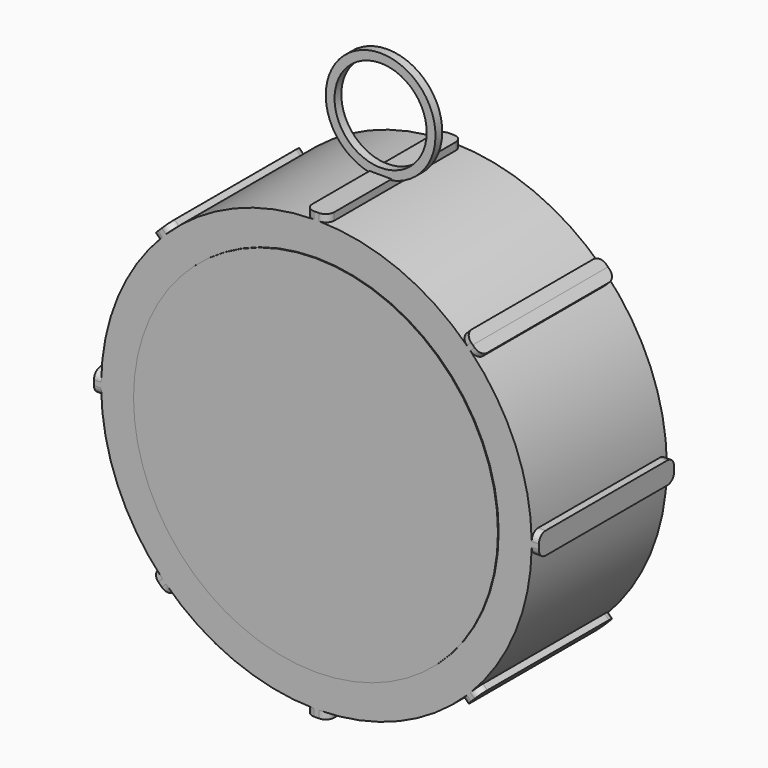
from build123d import *

# Parameters (mm, degrees)
F0_R     = 32.3708711279
F1_DEPTH = 12.7
F2_R     = 27.3986132433
F3_DEPTH = 12.827
F5_DEPTH = 25.4
F6_R     = 1.27
F8_R     = 8.2490124286
F8_R_2   = 6.9276952265
F9_DEPTH = 0.635


# Not quite as in the source:
# - two fillets or chamfers of one size are made in one step


with BuildPart() as f1:
    # F0 (on Front) → F1 (new body, symmetric)
    with BuildSketch(Plane.XZ):
        Circle(F0_R)
    extrude(amount=F1_DEPTH, both=True)

    # F2 (on Front) → F3 (join, symmetric)
    with BuildSketch(Plane.XZ):
        Circle(F2_R)
    extrude(amount=F3_DEPTH, both=True)

    # F4 (on face) → F5 (join)
    with BuildSketch(Plane.XZ.offset(12.7)):
        with BuildLine():
            ThreePointArc((-24.0273053052, 21.6924387138), (-22.8896624875, 22.8896624875), (-21.6924387138, 24.0273053052))
            Line((-21.6924387138, 24.0273053052), (-22.3403787647, 24.6752453562))
            Line((-22.3403787647, 24.6752453562), (-23.5078120604, 23.5078120604))
            Line((-23.5078120604, 23.5078120604), (-24.6752453562, 22.3403787647))
            Line((-24.6752453562, 22.3403787647), (-24.0273053052, 21.6924387138))
        make_face()
        with BuildLine():
            Line((24.6752453562, 22.3403787647), (23.5078120604, 23.5078120604))
            Line((23.5078120604, 23.5078120604), (22.3403787647, 24.6752453562))
            Line((22.3403787647, 24.6752453562), (21.6924387138, 24.0273053052))
            ThreePointArc((21.6924387138, 24.0273053052), (22.8896624875, 22.8896624875), (24.0273053052, 21.6924387138))
            Line((24.0273053052, 21.6924387138), (24.6752453562, 22.3403787647))
        make_face()
        with BuildLine():
            Line((24.6752453562, -22.3403787647), (24.0273053052, -21.6924387138))
            ThreePointArc((24.0273053052, -21.6924387138), (22.8896624875, -22.8896624875), (21.6924387138, -24.0273053052))
            Line((21.6924387138, -24.0273053052), (22.3403787647, -24.6752453562))
            Line((22.3403787647, -24.6752453562), (23.5078120604, -23.5078120604))
            Line((23.5078120604, -23.5078120604), (24.6752453562, -22.3403787647))
        make_face()
        with BuildLine():
            ThreePointArc((-21.6924387138, -24.0273053052), (-22.8896624875, -22.8896624875), (-24.0273053052, -21.6924387138))
            Line((-24.0273053052, -21.6924387138), (-24.6752453562, -22.3403787647))
            Line((-24.6752453562, -22.3403787647), (-23.5078120604, -23.5078120604))
            Line((-23.5078120604, -23.5078120604), (-22.3403787647, -24.6752453562))
            Line((-22.3403787647, -24.6752453562), (-21.6924387138, -24.0273053052))
        make_face()
        with BuildLine():
            Line((1.651, -33.4515422583), (1.651, -32.3287410299))
            ThreePointArc((1.651, -32.3287410299), (0, -32.3708711279), (-1.651, -32.3287410299))
            Line((-1.651, -32.3287410299), (-1.651, -33.4515422583))
            Line((-1.651, -33.4515422583), (0, -33.4515422583))
            Line((0, -33.4515422583), (1.651, -33.4515422583))
        make_face()
        with BuildLine():
            ThreePointArc((-32.3287410299, -1.651), (-32.3708711279, 0), (-32.3287410299, 1.651))
            Line((-32.3287410299, 1.651), (-33.4515480299, 1.651))
            Line((-33.4515480299, 1.651), (-33.4515480299, 0))
            Line((-33.4515480299, 0), (-33.4515480299, -1.651))
            Line((-33.4515480299, -1.651), (-32.3287410299, -1.651))
        make_face()
        with BuildLine():
            Line((33.4515480299, 1.651), (32.3287410299, 1.651))
            ThreePointArc((32.3287410299, 1.651), (32.3603368894, 0.8257687245), (32.3708711279, 0))
            ThreePointArc((32.3708711279, 0), (32.3603368894, -0.8257687245), (32.3287410299, -1.651))
            Line((32.3287410299, -1.651), (33.4515480299, -1.651))
            Line((33.4515480299, -1.651), (33.4515480299, 0))
            Line((33.4515480299, 0), (33.4515480299, 1.651))
        make_face()
        with BuildLine():
            ThreePointArc((-1.651, 32.3287410299), (0, 32.3708711279), (1.651, 32.3287410299))
            Line((1.651, 32.3287410299), (1.651, 33.4515422583))
            Line((1.651, 33.4515422583), (0, 33.4515422583))
            Line((0, 33.4515422583), (-1.651, 33.4515422583))
            Line((-1.651, 33.4515422583), (-1.651, 32.3287410299))
        make_face()
    extrude(amount=-F5_DEPTH)

    # F6
    f6_edges = [f1.edges().sort_by_distance(p)[0] for p in [
        (24.351275, 12.7, -22.016409),
        (22.016409, 12.7, -24.351275),
        (24.351275, -12.7, -22.016409),
        (22.016409, -12.7, -24.351275),
        (24.351275, -12.7, 22.016409),
        (22.016409, -12.7, 24.351275),
        (22.016409, 12.7, 24.351275),
        (24.351275, 12.7, 22.016409),
        (-22.016409, 12.7, 24.351275),
        (-24.351275, 12.7, 22.016409),
        (-24.351275, 12.7, -22.016409),
        (-22.016409, 12.7, -24.351275),
        (-22.016409, -12.7, -24.351275),
        (-24.351275, -12.7, -22.016409),
        (-24.351275, -12.7, 22.016409),
        (-22.016409, -12.7, 24.351275),
        (32.890145, -12.7, 1.651),
        (32.890145, 12.7, 1.651),
        (1.651, -12.7, 32.890142),
        (-1.651, -12.7, 32.890142),
        (-32.890145, -12.7, 1.651),
        (-32.890145, -12.7, -1.651),
        (-1.651, -12.7, -32.890142),
        (1.651, -12.7, -32.890142),
        (32.890145, -12.7, -1.651),
        (1.651, 12.7, 32.890142),
        (-1.651, 12.7, 32.890142),
        (-32.890145, 12.7, 1.651),
        (-32.890145, 12.7, -1.651),
        (-1.651, 12.7, -32.890142),
        (1.651, 12.7, -32.890142),
        (32.890145, 12.7, -1.651),
    ]]
    fillet(f6_edges, radius=F6_R)

    # F8 (on Front) → F9 (join, symmetric)
    with BuildSketch(Plane.XZ):
        with Locations((0, 41.3398481905)):
            Circle(F8_R)
        with Locations((0, 41.3398481905)):
            Circle(F8_R_2, mode=Mode.SUBTRACT)
    extrude(amount=F9_DEPTH, both=True)


solid = f1.part
